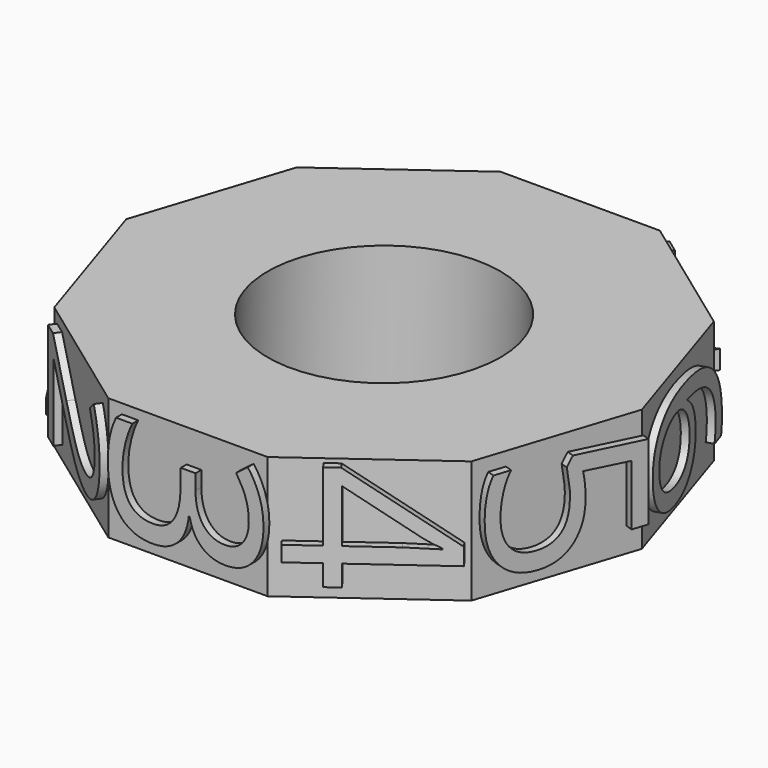
from build123d import *

# Parameters (mm, degrees)
F0_R          = 12.065
F1_DEPTH      = 12.7
F2_TEXT_SIZE  = 22.9248896787
F3_DEPTH      = 0.762
F4_TEXT_SIZE  = 21.7850442241
F5_DEPTH      = 0.762
F6_TEXT_SIZE  = 21.9735063531
F7_DEPTH      = 0.762
F8_TEXT_SIZE  = 20.598073999
F9_DEPTH      = 0.762
F10_TEXT_SIZE = 21.9320021587
F11_DEPTH     = 0.762
F12_TEXT_SIZE = 21.605528974
F13_DEPTH     = 0.762
F14_TEXT_SIZE = 21.6804481195
F15_DEPTH     = 0.762
F16_TEXT_SIZE = 21.7152017099
F17_DEPTH     = 0.762
F18_TEXT_SIZE = 21.7850442241
F19_DEPTH     = 0.762
F20_TEXT_SIZE = 21.6400425985
F21_DEPTH     = 0.762


# Not quite as in the source:
# - Text() gives the source's letters only with a copy of the font that has no kerning and outlines rounded to 1/6400 em; it was checked with that copy


with BuildPart() as f1:
    # F0 (on Top) → F1 (new body)
    with BuildSketch(Plane.XY):
        Polygon((8.2529602843, 25.4), (-8.2529602843, 25.4), (-21.6065305321, 15.6980633142), (-26.7071404957, 0), (-21.6065305321, -15.6980633142), (-8.2529602843, -25.4), (8.2529602843, -25.4), (21.6065305321, -15.6980633142), (26.7071404957, 0), (21.6065305321, 15.6980633142), align=None)
        Circle(F0_R, mode=Mode.SUBTRACT)
    extrude(amount=F1_DEPTH)

    # F2 (on face) → F3 (join)
    with BuildSketch(Plane(origin=(-24.1568355139, -7.8490316571, 0), x_dir=(0.3090169944, -0.9510565163, 0), z_dir=(-0.9510565163, -0.3090169944, 0))):
        with Locations(Location((-8.2529602843, 10.697556761), (0, 0, -90))):
            Text('1', F2_TEXT_SIZE, font='Open Sans', text_align=(TextAlign.LEFT, TextAlign.BOTTOM))
    extrude(amount=F3_DEPTH)

    # F4 (on face) → F5 (join)
    with BuildSketch(Plane(origin=(-14.9297454082, -20.5490316571, 0), x_dir=(0.8090169944, -0.5877852523, 0), z_dir=(-0.5877852523, -0.8090169944, 0))):
        with Locations(Location((-7.399420894, 12.7), (0, 0, -90))):
            Text('2', F4_TEXT_SIZE, font='Open Sans', text_align=(TextAlign.LEFT, TextAlign.BOTTOM))
    extrude(amount=F5_DEPTH)

    # F6 (on face) → F7 (join)
    with BuildSketch(Plane.XZ.offset(25.4)):
        with Locations(Location((-7.4753260273, 12.7), (0, 0, -90))):
            Text('3', F6_TEXT_SIZE, font='Open Sans', text_align=(TextAlign.LEFT, TextAlign.BOTTOM))
    extrude(amount=F7_DEPTH)

    # F8 (on face) → F9 (join)
    with BuildSketch(Plane(origin=(14.9297454082, -20.5490316571, 0), x_dir=(0.8090169944, 0.5877852523, 0), z_dir=(0.5877852523, -0.8090169944, 0))):
        with Locations(Location((-7.0992874923, 12.7), (0, 0, -90))):
            Text('4', F8_TEXT_SIZE, font='Open Sans', text_align=(TextAlign.LEFT, TextAlign.BOTTOM))
    extrude(amount=F9_DEPTH)

    # F10 (on face) → F11 (join)
    with BuildSketch(Plane(origin=(24.1568355139, -7.8490316571, 0), x_dir=(0.3090169944, 0.9510565163, 0), z_dir=(0.9510565163, -0.3090169944, 0))):
        with Locations(Location((-7.2559274406, 12.7), (0, 0, -90))):
            Text('5', F10_TEXT_SIZE, font='Open Sans', text_align=(TextAlign.LEFT, TextAlign.BOTTOM))
    extrude(amount=F11_DEPTH)

    # F12 (on face) → F13 (join)
    with BuildSketch(Plane(origin=(24.1568355139, 7.8490316571, 0), x_dir=(-0.3090169944, 0.9510565163, 0), z_dir=(0.9510565163, 0.3090169944, 0))):
        with Locations(Location((-7.5579203939, 12.7), (0, 0, -90))):
            Text('6', F12_TEXT_SIZE, font='Open Sans', text_align=(TextAlign.LEFT, TextAlign.BOTTOM))
    extrude(amount=F13_DEPTH)

    # F14 (on face) → F15 (join)
    with BuildSketch(Plane(origin=(14.9297454082, 20.5490316571, 0), x_dir=(-0.8090169944, 0.5877852523, 0), z_dir=(0.5877852523, 0.8090169944, 0))):
        with Locations(Location((-7.4127015932, 12.7), (0, 0, -90))):
            Text('7', F14_TEXT_SIZE, font='Open Sans', text_align=(TextAlign.LEFT, TextAlign.BOTTOM))
    extrude(amount=F15_DEPTH)

    # F16 (on face) → F17 (join)
    with BuildSketch(Plane(origin=(0, 25.4, 0), x_dir=(-1, 0, 0), z_dir=(0, 1, 0))):
        with Locations(Location((-8.2529602843, 12.7), (0, 0, -90))):
            Text('8', F16_TEXT_SIZE, font='Open Sans', text_align=(TextAlign.LEFT, TextAlign.BOTTOM))
    extrude(amount=F17_DEPTH)

    # F18 (on face) → F19 (join)
    with BuildSketch(Plane(origin=(-14.9297454082, 20.5490316571, 0), x_dir=(-0.8090169944, -0.5877852523, 0), z_dir=(-0.5877852523, 0.8090169944, 0))):
        with Locations(Location((-7.1690204391, 12.7), (0, 0, -90))):
            Text('9', F18_TEXT_SIZE, font='Open Sans', text_align=(TextAlign.LEFT, TextAlign.BOTTOM))
    extrude(amount=F19_DEPTH)

    # F20 (on face) → F21 (join)
    with BuildSketch(Plane(origin=(-24.1568355139, 7.8490316571, 0), x_dir=(-0.3090169944, -0.9510565163, 0), z_dir=(-0.9510565163, 0.3090169944, 0))):
        with Locations(Location((-7.1723343408, 12.7), (0, 0, -90))):
            Text('0', F20_TEXT_SIZE, font='Open Sans', text_align=(TextAlign.LEFT, TextAlign.BOTTOM))
    extrude(amount=F21_DEPTH)


solid = f1.part
